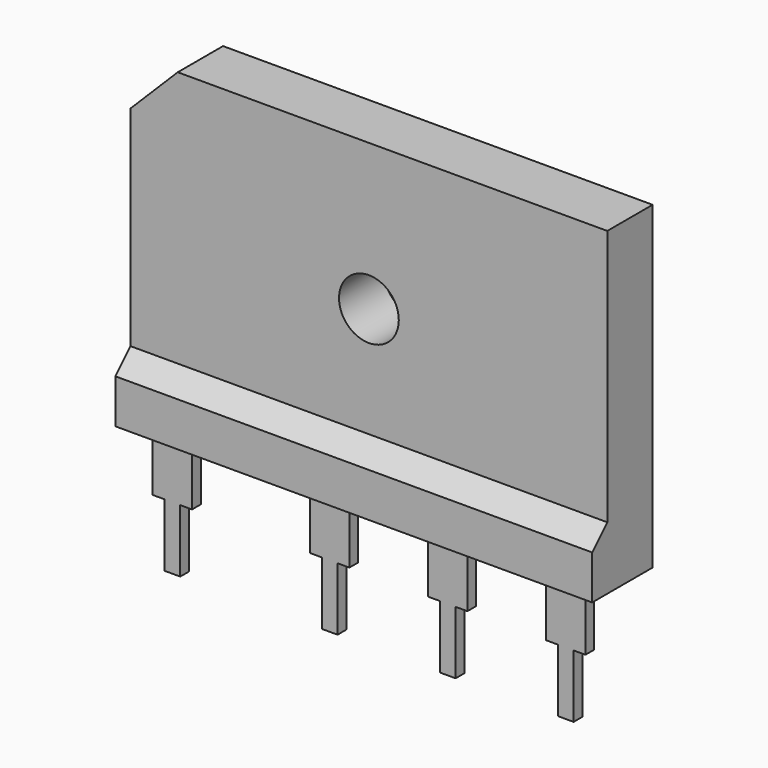
from build123d import *

# Parameters (mm, degrees)
F0_W     = 30.3
F0_H     = 20.3
F0_R     = 1.9
F1_DEPTH = 3.6
F2_W     = 30.3
F2_H     = 4
F3_DEPTH = 1.2
F4_SIZE  = 1.19999
F5_SIZE  = 3
F6_W     = 2.5
F6_H     = 0.7
F7_DEPTH = 4
F8_W     = 1
F8_H     = 0.7
F9_DEPTH = 4


# Not quite as in the source:
# - a fillet or chamfer is up to 0.001 mm smaller than in the source, because OpenCascade refuses the exact size


with BuildPart() as f1:
    # F0 (on Front) → F1 (new body)
    with BuildSketch(Plane.XZ):
        Rectangle(F0_W, F0_H)
        with Locations((0, 0.85)):
            Circle(F0_R, mode=Mode.SUBTRACT)
    extrude(amount=F1_DEPTH)

    # F2 (on face) → F3 (join)
    with BuildSketch(Plane.XZ.offset(3.6)):
        with Locations((0, -8.15)):
            Rectangle(F2_W, F2_H)
    extrude(amount=F3_DEPTH)

    # F4 (size 1.2 in the source; OpenCascade refuses exactly that, so slightly less here)
    f4_edges = [f1.edges().sort_by_distance(p)[0] for p in [
        (0, -4.8, -6.15),
    ]]
    chamfer(f4_edges, length=F4_SIZE)

    # F5
    f5_edges = [f1.edges().sort_by_distance(p)[0] for p in [
        (-15.15, -1.8, 10.15),
    ]]
    chamfer(f5_edges, length=F5_SIZE)


with BuildPart() as f7:
    # F6 (on face) → F7 (new body)
    with BuildSketch(Plane(origin=(0, 0, -10.15), x_dir=(1, 0, 0), z_dir=(0, 0, -1))):
        with Locations((-12.65, 3.05)):
            Rectangle(F6_W, F6_H)
    extrude(amount=F7_DEPTH)

    # F8 (on face) → F9 (join)
    with BuildSketch(Plane(origin=(0, 0, -14.15), x_dir=(1, 0, 0), z_dir=(0, 0, -1))):
        with Locations((-12.65, 3.05)):
            Rectangle(F8_W, F8_H)
    extrude(amount=F9_DEPTH)


with BuildPart() as f7b:
    # F6 (on face) → F7, piece 2 (new body)
    with BuildSketch(Plane(origin=(0, 0, -10.15), x_dir=(1, 0, 0), z_dir=(0, 0, -1))):
        with Locations((4.85, 3.05)):
            Rectangle(F6_W, F6_H)
    extrude(amount=F7_DEPTH)

    # F8 (on face) → F9, piece 3 (join)
    with BuildSketch(Plane(origin=(0, 0, -14.15), x_dir=(1, 0, 0), z_dir=(0, 0, -1))):
        with Locations((4.85, 3.05)):
            Rectangle(F8_W, F8_H)
    extrude(amount=F9_DEPTH)


with BuildPart() as f7c:
    # F6 (on face) → F7, piece 3 (new body)
    with BuildSketch(Plane(origin=(0, 0, -10.15), x_dir=(1, 0, 0), z_dir=(0, 0, -1))):
        with Locations((12.35, 3.05)):
            Rectangle(F6_W, F6_H)
    extrude(amount=F7_DEPTH)

    # F8 (on face) → F9, piece 4 (join)
    with BuildSketch(Plane(origin=(0, 0, -14.15), x_dir=(1, 0, 0), z_dir=(0, 0, -1))):
        with Locations((12.35, 3.05)):
            Rectangle(F8_W, F8_H)
    extrude(amount=F9_DEPTH)


with BuildPart() as f7d:
    # F6 (on face) → F7, piece 4 (new body)
    with BuildSketch(Plane(origin=(0, 0, -10.15), x_dir=(1, 0, 0), z_dir=(0, 0, -1))):
        with Locations((-2.65, 3.05)):
            Rectangle(F6_W, F6_H)
    extrude(amount=F7_DEPTH)

    # F8 (on face) → F9, piece 2 (join)
    with BuildSketch(Plane(origin=(0, 0, -14.15), x_dir=(1, 0, 0), z_dir=(0, 0, -1))):
        with Locations((-2.65, 3.05)):
            Rectangle(F8_W, F8_H)
    extrude(amount=F9_DEPTH)


solid = Compound([f1.part, f7.part, f7b.part, f7c.part, f7d.part])
